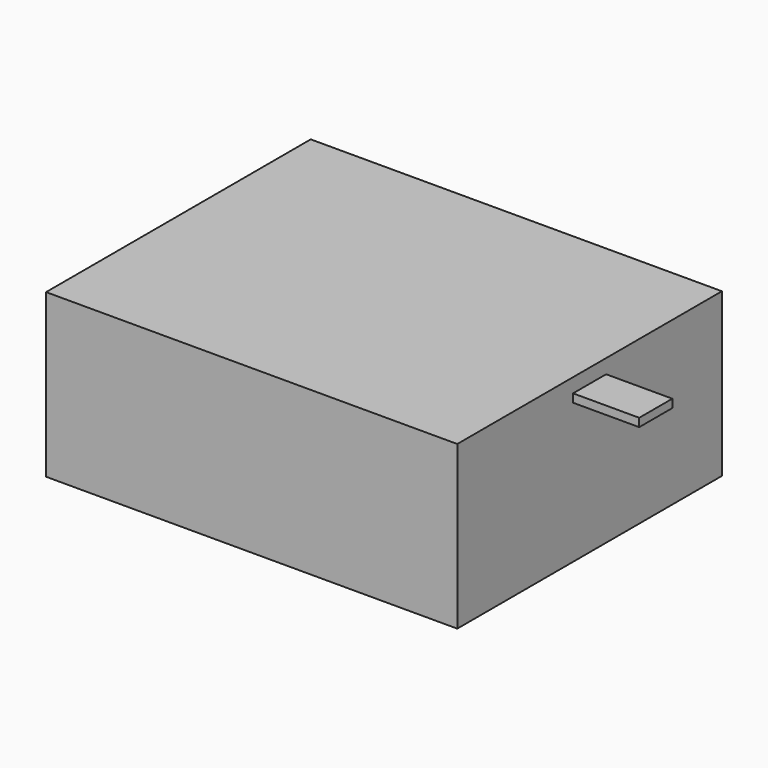
from build123d import *

# Parameters (mm, degrees)
F0_W     = 63.144043088
F0_H     = 24.9639227986
F1_DEPTH = 25.4
F2_W     = 10.16
F2_H     = 1.27
F3_DEPTH = 3.175
F4_W     = 10.16
F4_H     = 1.27
F5_DEPTH = 3.175


# Not quite as in the source:
# - a feature names something its author has since deleted; it is built from what else it names


with BuildPart() as f1:
    # F0 (on Front) → F1 (new body, symmetric)
    with BuildSketch(Plane.XZ):
        Rectangle(F0_W, F0_H)
    extrude(amount=F1_DEPTH, both=True)

    # F2 (on Front) → F3 (join, symmetric)
    with BuildSketch(Plane.XZ):
        with Locations((36.6514939815, 9.6600476645)):
            Rectangle(F2_W, F2_H)
    extrude(amount=F3_DEPTH, both=True)

    # F4 (on Front) → F5 (join, symmetric)
    with BuildSketch(Plane.XZ):
        with Locations((-36.6476550698, -9.8343824477)):
            Rectangle(F4_W, F4_H)
    extrude(amount=F5_DEPTH, both=True)


solid = f1.part
